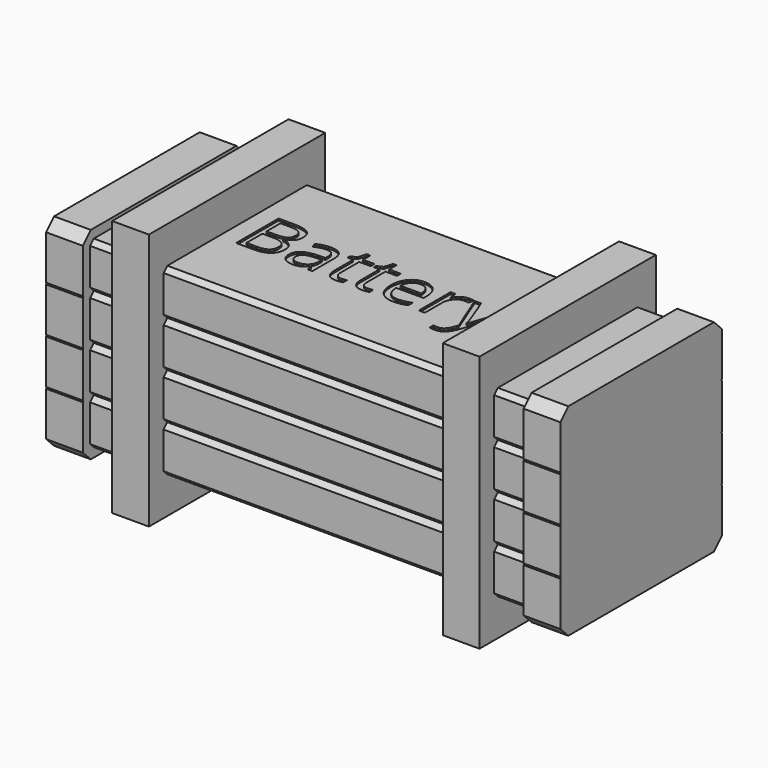
from build123d import *

# Parameters (mm, degrees)
F0_W          = 80
F0_H          = 100
F1_DEPTH      = 25
F2_SIZE       = 2.5
F5_W          = 120
F5_H          = 140
F6_DEPTH      = 10
F9_W          = 137.4242957681
F9_H          = 143.3767583221
F10_DEPTH     = 150
F12_W         = 132.6489392668
F12_H         = 149.268520996
F13_DEPTH     = 180
F15_DEPTH     = 20
F17_DEPTH     = 20
F18_TEXT_SIZE = 40.4612730361
F19_DEPTH     = 1


# Not quite as in the source:
# - Text() gives the source's letters only with a copy of the font that has no kerning and outlines rounded to 1/6400 em; it was checked with that copy


with BuildPart() as f1:
    # F0 (on Top) → F1 (new body)
    with BuildSketch(Plane.XY):
        with Locations((40, 50)):
            Rectangle(F0_W, F0_H)
    extrude(amount=F1_DEPTH)

    # F2
    f2_edges = [f1.edges().sort_by_distance(p)[0] for p in [
        (40, 0, 25),
        (40, 0, 0),
        (40, 100, 25),
        (40, 100, 0),
    ]]
    chamfer(f2_edges, length=F2_SIZE)

    # F3: F1 across face


with BuildPart() as f1_1:
    add(f1.part)
    add(f1.part.mirror(Plane(origin=(40, 50, 25), x_dir=(1, 0, 0), z_dir=(0, 0, 1))))

    # F4: F1 across face


with BuildPart() as f1_2:
    add(f1_1.part)
    add(f1_1.part.mirror(Plane(origin=(40, 50, 50), x_dir=(1, 0, 0), z_dir=(0, 0, 1))))

    # F5 (on face) → F6 (join)
    with BuildSketch(Plane.YZ.offset(80)):
        with Locations((50, 50)):
            Rectangle(F5_W, F5_H)
        Polygon((0, 2.5), (0, 22.5), (2.5, 25), (0, 27.5), (0, 47.5), (2.5, 50), (0, 52.5), (0, 72.5), (2.5, 75), (0, 77.5), (0, 97.5), (2.5, 100), (97.5, 100), (100, 97.5), (100, 77.5), (97.5, 75), (100, 72.5), (100, 52.5), (97.5, 50), (100, 47.5), (100, 27.5), (97.5, 25), (100, 22.5), (100, 2.5), (97.5, 0), (2.5, 0), align=None, mode=Mode.SUBTRACT)
        Polygon((2.5, 25), (0, 22.5), (0, 2.5), (2.5, 0), (97.5, 0), (100, 2.5), (100, 22.5), (97.5, 25), (100, 27.5), (100, 47.5), (97.5, 50), (100, 52.5), (100, 72.5), (97.5, 75), (100, 77.5), (100, 97.5), (97.5, 100), (2.5, 100), (0, 97.5), (0, 77.5), (2.5, 75), (0, 72.5), (0, 52.5), (2.5, 50), (0, 47.5), (0, 27.5), align=None)
    extrude(amount=F6_DEPTH)

    # F7: F1 across face


with BuildPart() as f1_3:
    add(f1_2.part)
    add(f1_2.part.mirror(Plane(origin=(0, 50, 50), x_dir=(0, -1, 0), z_dir=(-1, 0, 0))))

    # F8: F1 across face


with BuildPart() as f1_4:
    add(f1_3.part)
    add(f1_3.part.mirror(Plane(origin=(90, 50, 50), x_dir=(0, 1, 0), z_dir=(1, 0, 0))))

    # F9 (on face) → F10 (cut)
    with BuildSketch(Plane.YZ.offset(270)):
        with Locations((50.0000016764, 49.8705999926)):
            Rectangle(F9_W, F9_H)
    extrude(amount=-F10_DEPTH, mode=Mode.SUBTRACT)

    # F11: F1 across face


with BuildPart() as f1_5:
    add(f1_4.part)
    add(f1_4.part.mirror(Plane(origin=(-90, 50, 50), x_dir=(0, -1, 0), z_dir=(-1, 0, 0))))

    # F12 (on face) → F13 (cut)
    with BuildSketch(Plane(origin=(-300, 0, 0), x_dir=(0, -1, 0), z_dir=(-1, 0, 0))):
        with Locations((-49.6218679473, 49.5881671086)):
            Rectangle(F12_W, F12_H)
    extrude(amount=-F13_DEPTH, mode=Mode.SUBTRACT)

    # F14 (on face) → F15 (join)
    with BuildSketch(Plane.YZ.offset(120)):
        Polygon((104.5710631757, 25), (104.9999967217, 25.428933546), (104.9999967217, 49.571066454), (104.5710631757, 50), (104.9999967217, 50.428933546), (104.9999967217, 74.571066454), (104.5710631757, 75), (104.9999967217, 75.428933546), (104.9999967217, 99.571066454), (99.571066454, 104.9999967217), (0.428933546, 104.9999967217), (-4.9999967217, 99.571066454), (-4.9999967217, 75.428933546), (-4.5710631757, 75), (-4.9999967217, 74.571066454), (-4.9999967217, 50.428933546), (-4.5710631757, 50), (-4.9999967217, 49.571066454), (-4.9999967217, 25.428933546), (-4.5710631757, 25), (-4.9999967217, 24.571066454), (-4.9999967217, 0.428933546), (0.428933546, -4.9999967217), (99.571066454, -4.9999967217), (104.9999967217, 0.428933546), (104.9999967217, 24.571066454), align=None)
        Polygon((100, 2.5), (97.5, 0), (2.5, 0), (0, 2.5), (0, 22.5), (2.5, 25), (0, 27.5), (0, 47.5), (2.5, 50), (0, 52.5), (0, 72.5), (2.5, 75), (0, 77.5), (0, 97.5), (2.5, 100), (97.5, 100), (100, 97.5), (100, 77.5), (97.5, 75), (100, 72.5), (100, 52.5), (97.5, 50), (100, 47.5), (100, 27.5), (97.5, 25), (100, 22.5), align=None, mode=Mode.SUBTRACT)
        Polygon((2.5, 0), (97.5, 0), (100, 2.5), (100, 22.5), (97.5, 25), (100, 27.5), (100, 47.5), (97.5, 50), (100, 52.5), (100, 72.5), (97.5, 75), (100, 77.5), (100, 97.5), (97.5, 100), (2.5, 100), (0, 97.5), (0, 77.5), (2.5, 75), (0, 72.5), (0, 52.5), (2.5, 50), (0, 47.5), (0, 27.5), (2.5, 25), (0, 22.5), (0, 2.5), align=None)
    extrude(amount=F15_DEPTH)

    # F16 (on face) → F17 (join)
    with BuildSketch(Plane(origin=(-120, 0, 0), x_dir=(0, -1, 0), z_dir=(-1, 0, 0))):
        Polygon((-104.5710678119, 25), (-105, 24.5710678119), (-105, 0.4289321881), (-99.5710678119, -5), (-0.4289321881, -5), (5, 0.4289321881), (5, 24.5710678119), (4.5710678119, 25), (5, 25.4289321881), (5, 49.5710678119), (4.5710678119, 50), (5, 50.4289321881), (5, 74.5710678119), (4.5710678119, 75), (5, 75.4289321881), (5, 99.5710678119), (-0.4289321881, 105), (-99.5710678119, 105), (-105, 99.5710678119), (-105, 75.4289321881), (-104.5710678119, 75), (-105, 74.5710678119), (-105, 50.4289321881), (-104.5710678119, 50), (-105, 49.5710678119), (-105, 25.4289321881), align=None)
    extrude(amount=F17_DEPTH)

    # F18 (on face) → F19 (cut)
    with BuildSketch(Plane.XY.offset(100)):
        with Locations((-74.1697028279, 37.1082015336)):
            Text('Battery', F18_TEXT_SIZE, font='Open Sans', text_align=(TextAlign.LEFT, TextAlign.BOTTOM))
    extrude(amount=-F19_DEPTH, mode=Mode.SUBTRACT)


solid = f1_5.part
